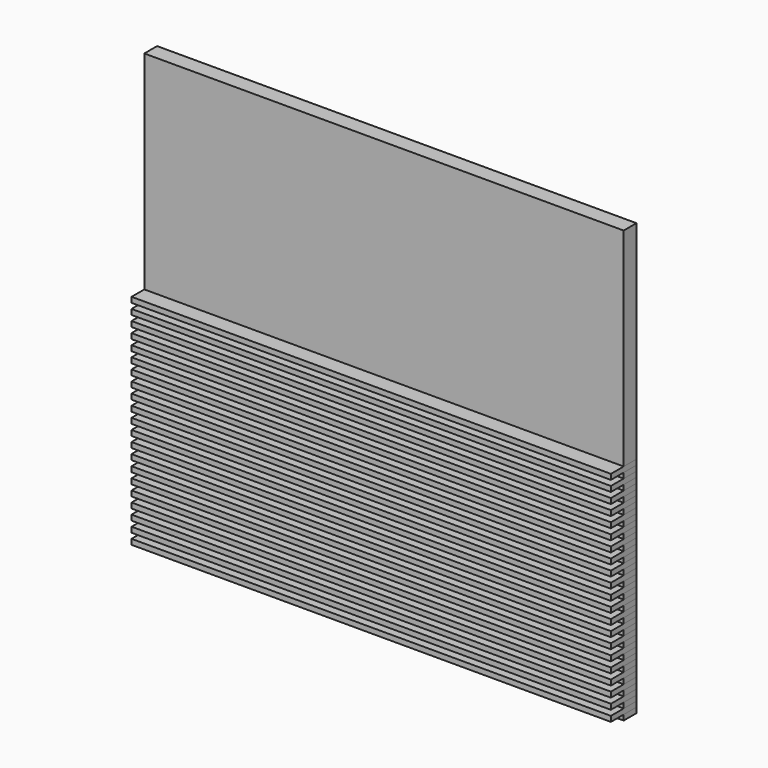
from build123d import *

# Parameters (mm, degrees)
F0_W     = 571.5
F0_H     = 6.35
F1_DEPTH = 38.1
F0_H_2   = 241.3
F2_DEPTH = 19.05


# Not quite as in the source:
# - a feature names something its author has since deleted; it is built from what else it names


with BuildPart() as f1:
    # F0 (on Front) → F1 (new body)
    with BuildSketch(Plane.XZ):
        with Locations((-27.4516956389, -70.8882805049)):
            Rectangle(F0_W, F0_H)
    extrude(amount=F1_DEPTH)


with BuildPart() as f1b:
    # F0 (on Front) → F1, piece 2 (new body)
    with BuildSketch(Plane.XZ):
        with Locations((-27.4516956389, -45.4882805049)):
            Rectangle(F0_W, F0_H)
    extrude(amount=F1_DEPTH)


with BuildPart() as f1c:
    # F0 (on Front) → F1, piece 3 (new body)
    with BuildSketch(Plane.XZ):
        with Locations((-27.4516956389, 5.3117194951)):
            Rectangle(F0_W, F0_H)
    extrude(amount=F1_DEPTH)


with BuildPart() as f1d:
    # F0 (on Front) → F1, piece 4 (new body)
    with BuildSketch(Plane.XZ):
        with Locations((-27.4516956389, -58.1882805049)):
            Rectangle(F0_W, F0_H)
    extrude(amount=F1_DEPTH)


with BuildPart() as f1e:
    # F0 (on Front) → F1, piece 5 (new body)
    with BuildSketch(Plane.XZ):
        with Locations((-27.4516956389, -32.7882805049)):
            Rectangle(F0_W, F0_H)
    extrude(amount=F1_DEPTH)


with BuildPart() as f1f:
    # F0 (on Front) → F1, piece 6 (new body)
    with BuildSketch(Plane.XZ):
        with Locations((-27.4516956389, -20.0882805049)):
            Rectangle(F0_W, F0_H)
    extrude(amount=F1_DEPTH)


with BuildPart() as f1g:
    # F0 (on Front) → F1, piece 7 (new body)
    with BuildSketch(Plane.XZ):
        with Locations((-27.4516956389, -7.3882805049)):
            Rectangle(F0_W, F0_H)
    extrude(amount=F1_DEPTH)


with BuildPart() as f1h:
    # F0 (on Front) → F1, piece 8 (new body)
    with BuildSketch(Plane.XZ):
        with Locations((-27.4516956389, 18.0117194951)):
            Rectangle(F0_W, F0_H)
    extrude(amount=F1_DEPTH)


with BuildPart() as f1i:
    # F0 (on Front) → F1, piece 9 (new body)
    with BuildSketch(Plane.XZ):
        with Locations((-27.4516956389, 30.7117194951)):
            Rectangle(F0_W, F0_H)
    extrude(amount=F1_DEPTH)


with BuildPart() as f1j:
    # F0 (on Front) → F1, piece 10 (new body)
    with BuildSketch(Plane.XZ):
        with Locations((-27.4516956389, 43.4117194951)):
            Rectangle(F0_W, F0_H)
    extrude(amount=F1_DEPTH)


with BuildPart() as f1k:
    # F0 (on Front) → F1, piece 11 (new body)
    with BuildSketch(Plane.XZ):
        with Locations((-27.4516956389, 56.1117194951)):
            Rectangle(F0_W, F0_H)
    extrude(amount=F1_DEPTH)


with BuildPart() as f1l:
    # F0 (on Front) → F1, piece 12 (new body)
    with BuildSketch(Plane.XZ):
        with Locations((-27.4516956389, 68.8117194951)):
            Rectangle(F0_W, F0_H)
    extrude(amount=F1_DEPTH)


with BuildPart() as f1m:
    # F0 (on Front) → F1, piece 13 (new body)
    with BuildSketch(Plane.XZ):
        with Locations((-27.4516956389, 81.5117194951)):
            Rectangle(F0_W, F0_H)
    extrude(amount=F1_DEPTH)


with BuildPart() as f1n:
    # F0 (on Front) → F1, piece 14 (new body)
    with BuildSketch(Plane.XZ):
        with Locations((-27.4516956389, 94.2117194951)):
            Rectangle(F0_W, F0_H)
    extrude(amount=F1_DEPTH)


with BuildPart() as f1o:
    # F0 (on Front) → F1, piece 15 (new body)
    with BuildSketch(Plane.XZ):
        with Locations((-27.4516956389, 106.9117194951)):
            Rectangle(F0_W, F0_H)
    extrude(amount=F1_DEPTH)


with BuildPart() as f1p:
    # F0 (on Front) → F1, piece 16 (new body)
    with BuildSketch(Plane.XZ):
        with Locations((-27.4516956389, 119.6117194951)):
            Rectangle(F0_W, F0_H)
    extrude(amount=F1_DEPTH)


with BuildPart() as f1q:
    # F0 (on Front) → F1, piece 17 (new body)
    with BuildSketch(Plane.XZ):
        with Locations((-27.4516956389, 132.3117194951)):
            Rectangle(F0_W, F0_H)
    extrude(amount=F1_DEPTH)


with BuildPart() as f1r:
    # F0 (on Front) → F1, piece 18 (new body)
    with BuildSketch(Plane.XZ):
        with Locations((-27.4516956389, 145.0117194951)):
            Rectangle(F0_W, F0_H)
    extrude(amount=F1_DEPTH)


with BuildPart() as f1s:
    # F0 (on Front) → F1, piece 19 (new body)
    with BuildSketch(Plane.XZ):
        with Locations((-27.4516956389, 157.7117194951)):
            Rectangle(F0_W, F0_H)
    extrude(amount=F1_DEPTH)


with BuildPart() as f1t:
    # F0 (on Front) → F1, piece 20 (new body)
    with BuildSketch(Plane.XZ):
        with Locations((-27.4516956389, -83.5882805049)):
            Rectangle(F0_W, F0_H)
    extrude(amount=F1_DEPTH)


with BuildPart() as f1u:
    # F0 (on Front) → F1, piece 21 (new body)
    with BuildSketch(Plane.XZ):
        with Locations((-27.4516956389, -96.2882805049)):
            Rectangle(F0_W, F0_H)
    extrude(amount=F1_DEPTH)


with BuildPart() as f2:
    # F0 (on Front) → F2 (new body)
    with BuildSketch(Plane.XZ):
        with Locations((-27.4516956389, 164.0617194951)):
            Rectangle(F0_W, F0_H)
        with Locations((-27.4516956389, 287.8867194951)):
            Rectangle(F0_W, F0_H_2)
    extrude(amount=F2_DEPTH)


with BuildPart() as f2b:
    # F0 (on Front) → F2, piece 2 (new body)
    with BuildSketch(Plane.XZ):
        with Locations((-27.4516956389, 151.3617194951)):
            Rectangle(F0_W, F0_H)
    extrude(amount=F2_DEPTH)


with BuildPart() as f2c:
    # F0 (on Front) → F2, piece 3 (new body)
    with BuildSketch(Plane.XZ):
        with Locations((-27.4516956389, 138.6617194951)):
            Rectangle(F0_W, F0_H)
    extrude(amount=F2_DEPTH)


with BuildPart() as f2d:
    # F0 (on Front) → F2, piece 4 (new body)
    with BuildSketch(Plane.XZ):
        with Locations((-27.4516956389, 125.9617194951)):
            Rectangle(F0_W, F0_H)
    extrude(amount=F2_DEPTH)


with BuildPart() as f2e:
    # F0 (on Front) → F2, piece 5 (new body)
    with BuildSketch(Plane.XZ):
        with Locations((-27.4516956389, 113.2617194951)):
            Rectangle(F0_W, F0_H)
    extrude(amount=F2_DEPTH)


with BuildPart() as f2f:
    # F0 (on Front) → F2, piece 6 (new body)
    with BuildSketch(Plane.XZ):
        with Locations((-27.4516956389, 100.5617194951)):
            Rectangle(F0_W, F0_H)
    extrude(amount=F2_DEPTH)


with BuildPart() as f2g:
    # F0 (on Front) → F2, piece 7 (new body)
    with BuildSketch(Plane.XZ):
        with Locations((-27.4516956389, 87.8617194951)):
            Rectangle(F0_W, F0_H)
    extrude(amount=F2_DEPTH)


with BuildPart() as f2h:
    # F0 (on Front) → F2, piece 8 (new body)
    with BuildSketch(Plane.XZ):
        with Locations((-27.4516956389, 75.1617194951)):
            Rectangle(F0_W, F0_H)
    extrude(amount=F2_DEPTH)


with BuildPart() as f2i:
    # F0 (on Front) → F2, piece 9 (new body)
    with BuildSketch(Plane.XZ):
        with Locations((-27.4516956389, 62.4617194951)):
            Rectangle(F0_W, F0_H)
    extrude(amount=F2_DEPTH)


with BuildPart() as f2j:
    # F0 (on Front) → F2, piece 10 (new body)
    with BuildSketch(Plane.XZ):
        with Locations((-27.4516956389, 49.7617194951)):
            Rectangle(F0_W, F0_H)
    extrude(amount=F2_DEPTH)


with BuildPart() as f2k:
    # F0 (on Front) → F2, piece 11 (new body)
    with BuildSketch(Plane.XZ):
        with Locations((-27.4516956389, 37.0617194951)):
            Rectangle(F0_W, F0_H)
    extrude(amount=F2_DEPTH)


with BuildPart() as f2l:
    # F0 (on Front) → F2, piece 12 (new body)
    with BuildSketch(Plane.XZ):
        with Locations((-27.4516956389, 24.3617194951)):
            Rectangle(F0_W, F0_H)
    extrude(amount=F2_DEPTH)


with BuildPart() as f2m:
    # F0 (on Front) → F2, piece 13 (new body)
    with BuildSketch(Plane.XZ):
        with Locations((-27.4516956389, 11.6617194951)):
            Rectangle(F0_W, F0_H)
    extrude(amount=F2_DEPTH)


with BuildPart() as f2n:
    # F0 (on Front) → F2, piece 14 (new body)
    with BuildSketch(Plane.XZ):
        with Locations((-27.4516956389, -1.0382805049)):
            Rectangle(F0_W, F0_H)
    extrude(amount=F2_DEPTH)


with BuildPart() as f2o:
    # F0 (on Front) → F2, piece 15 (new body)
    with BuildSketch(Plane.XZ):
        with Locations((-27.4516956389, -13.7382805049)):
            Rectangle(F0_W, F0_H)
    extrude(amount=F2_DEPTH)


with BuildPart() as f2p:
    # F0 (on Front) → F2, piece 16 (new body)
    with BuildSketch(Plane.XZ):
        with Locations((-27.4516956389, -26.4382805049)):
            Rectangle(F0_W, F0_H)
    extrude(amount=F2_DEPTH)


with BuildPart() as f2q:
    # F0 (on Front) → F2, piece 17 (new body)
    with BuildSketch(Plane.XZ):
        with Locations((-27.4516956389, -39.1382805049)):
            Rectangle(F0_W, F0_H)
    extrude(amount=F2_DEPTH)


with BuildPart() as f2r:
    # F0 (on Front) → F2, piece 18 (new body)
    with BuildSketch(Plane.XZ):
        with Locations((-27.4516956389, -51.8382805049)):
            Rectangle(F0_W, F0_H)
    extrude(amount=F2_DEPTH)


with BuildPart() as f2s:
    # F0 (on Front) → F2, piece 19 (new body)
    with BuildSketch(Plane.XZ):
        with Locations((-27.4516956389, -64.5382805049)):
            Rectangle(F0_W, F0_H)
    extrude(amount=F2_DEPTH)


with BuildPart() as f2t:
    # F0 (on Front) → F2, piece 20 (new body)
    with BuildSketch(Plane.XZ):
        with Locations((-27.4516956389, -77.2382805049)):
            Rectangle(F0_W, F0_H)
    extrude(amount=F2_DEPTH)


with BuildPart() as f2u:
    # F0 (on Front) → F2, piece 21 (new body)
    with BuildSketch(Plane.XZ):
        with Locations((-27.4516956389, -89.9382805049)):
            Rectangle(F0_W, F0_H)
    extrude(amount=F2_DEPTH)


with BuildPart() as f2v:
    # F0 (on Front) → F2, piece 22 (new body)
    with BuildSketch(Plane.XZ):
        with Locations((-27.4516956389, -102.6382805049)):
            Rectangle(F0_W, F0_H)
    extrude(amount=F2_DEPTH)


solid = Compound([f1.part, f1b.part, f1c.part, f1d.part, f1e.part, f1f.part, f1g.part, f1h.part, f1i.part, f1j.part, f1k.part, f1l.part, f1m.part, f1n.part, f1o.part, f1p.part, f1q.part, f1r.part, f1s.part, f1t.part, f1u.part, f2.part, f2b.part, f2c.part, f2d.part, f2e.part, f2f.part, f2g.part, f2h.part, f2i.part, f2j.part, f2k.part, f2l.part, f2m.part, f2n.part, f2o.part, f2p.part, f2q.part, f2r.part, f2s.part, f2t.part, f2u.part, f2v.part])
